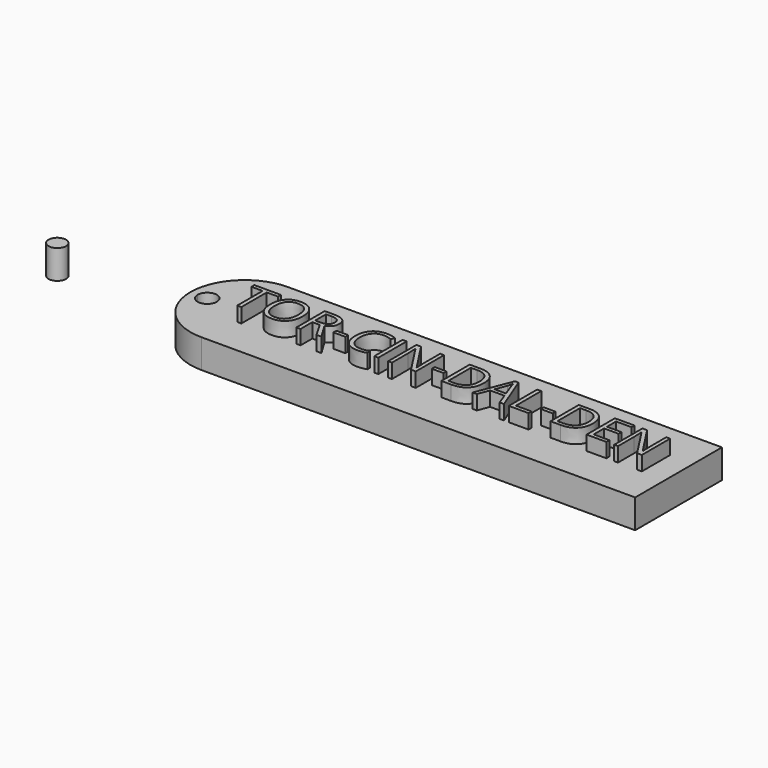
from build123d import *

# Parameters (mm, degrees)
F1_TEXT_SIZE = 8.7010705057
F2_DEPTH     = 2.54
F3_DEPTH     = 5.08
F0_R         = 1.5389917731


# Not quite as in the source:
# - Text() gives the source's letters only with a copy of the font that has no kerning and outlines rounded to 1/6400 em; it was checked with that copy


with BuildPart() as f2:
    # F1 (on Top) → F2 (new body)
    with BuildSketch(Plane.XY):
        with Locations((-21.9925081907, -2.920044432)):
            Text('TOR-CIN-DAL-DEN', F1_TEXT_SIZE, font='Open Sans', text_align=(TextAlign.LEFT, TextAlign.BOTTOM))
    extrude(amount=F2_DEPTH)


with BuildPart() as f3:
    # F0 (on Top) → F3 (new body)
    with BuildSketch(Plane.XY):
        Polygon((55.2200237185, -9.525), (55.2200237185, 9.525), (-20.9799762815, 9.525), (-20.9799762815, 0), (-20.9799762815, -9.525), align=None)
        with BuildLine():
            Line((-20.9799762815, 0), (-20.9799762815, 9.525))
            ThreePointArc((-20.9799762815, 9.525), (-27.7151683723, 6.7351920908), (-30.5049762815, 0))
            Line((-30.5049762815, 0), (-29.2343582808, 0))
            ThreePointArc((-29.2343582808, 0), (-27.555687353, 1.6786709278), (-25.8770164253, 0))
            Line((-25.8770164253, 0), (-20.9799762815, 0))
        make_face()
        with BuildLine():
            Line((-20.9799762815, -9.525), (-20.9799762815, 0))
            Line((-20.9799762815, 0), (-25.8770164253, 0))
            ThreePointArc((-25.8770164253, 0), (-27.555687353, -1.6786709278), (-29.2343582808, 0))
            Line((-29.2343582808, 0), (-30.5049762815, 0))
            ThreePointArc((-30.5049762815, 0), (-27.7151683723, -6.7351920908), (-20.9799762815, -9.525))
        make_face()
    extrude(amount=-F3_DEPTH)


with BuildPart() as f3b:
    # F0 (on Top) → F3, piece 2 (new body)
    with BuildSketch(Plane.XY):
        with Locations((-53.8912899792, 0)):
            Circle(F0_R)
    extrude(amount=-F3_DEPTH)


solid = Compound([f2.part, f3.part, f3b.part])
